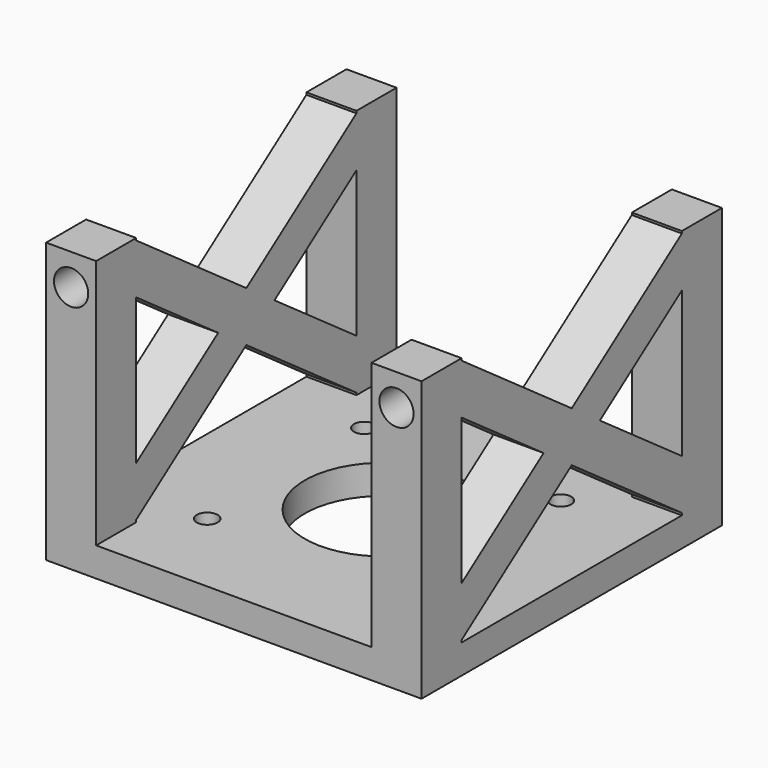
from build123d import *

# Parameters (mm, degrees)
F0_W      = 90
F0_H      = 90
F0_R      = 2.5
F0_R_2    = 19
F1_DEPTH  = 7
F3_W      = 12
F3_H      = 12
F4_DEPTH  = 60
F6_R      = 4.1
F7_DEPTH  = 100
F8_DEPTH  = 25
F12_DEPTH = 12
F15_DEPTH = 12


with BuildPart() as f1:
    # F0 (on Top) → F1 (new body)
    with BuildSketch(Plane.XY):
        Rectangle(F0_W, F0_H)
        with Locations((-23.55, -23.55)):
            Circle(F0_R, mode=Mode.SUBTRACT)
        with Locations((23.55, -23.55)):
            Circle(F0_R, mode=Mode.SUBTRACT)
        with Locations((-23.55, 23.55)):
            Circle(F0_R, mode=Mode.SUBTRACT)
        Circle(F0_R_2, mode=Mode.SUBTRACT)
        with Locations((23.55, 23.55)):
            Circle(F0_R, mode=Mode.SUBTRACT)
    extrude(amount=F1_DEPTH)

    # F3 (on offset) → F4 (join)
    with BuildSketch(Plane.XY.offset(7)):
        with Locations((-39, 39)):
            Rectangle(F3_W, F3_H)
        with Locations((39, 39)):
            Rectangle(F3_W, F3_H)
        with Locations((39, -39)):
            Rectangle(F3_W, F3_H)
        with Locations((-39, -39)):
            Rectangle(F3_W, F3_H)
    extrude(amount=F4_DEPTH)

    # F6 (on offset) → F7 (cut)
    with BuildSketch(Plane.XZ.offset(45)):
        with Locations((-39, 59.5)):
            Circle(F6_R)
        with Locations((39, 59.5)):
            Circle(F6_R)
    extrude(amount=-F7_DEPTH, mode=Mode.SUBTRACT)

    # F0 (on Top) → F8 (cut)
    with BuildSketch(Plane.XY):
        Circle(F0_R_2)
        with Locations((-23.55, 23.55)):
            Circle(F0_R)
        with Locations((23.55, 23.55)):
            Circle(F0_R)
        with Locations((23.55, -23.55)):
            Circle(F0_R)
        with Locations((-23.55, -23.55)):
            Circle(F0_R)
    extrude(amount=-F8_DEPTH, mode=Mode.SUBTRACT)

    # F11 (on face) → F12 (join)
    with BuildSketch(Plane.YZ.offset(45)):
        Polygon((0, 43), (-33, 66.4730164111), (-33, 54.4730164111), (-8.4352175508, 37), align=None)
        Polygon((33, 66.4730164111), (0, 43), (8.4352175508, 37), (33, 54.4730164111), align=None)
        Polygon((33, 19.5269835889), (8.4352175508, 37), (0, 31), (33, 7.5269835889), align=None)
        Polygon((0, 31), (-8.4352175508, 37), (-33, 19.5269835889), (-33, 7.5269835889), align=None)
        Polygon((8.4352175508, 37), (0, 43), (-8.4352175508, 37), (0, 31), align=None)
    extrude(amount=-F12_DEPTH)

    # F14 (on offset) → F15 (join)
    with BuildSketch(Plane(origin=(-45, 0, 0), x_dir=(0, -1, 0), z_dir=(-1, 0, 0))):
        Polygon((0, 43), (-33, 66.4730164111), (-33, 54.4730164111), (-8.4352175508, 37), (-33, 19.5269835889), (-33, 7.5269835889), (0, 31), (33, 7.5269835889), (33, 19.5269835889), (8.4352175508, 37), (33, 54.4730164111), (33, 66.4730164111), align=None)
    extrude(amount=-F15_DEPTH)


solid = f1.part
